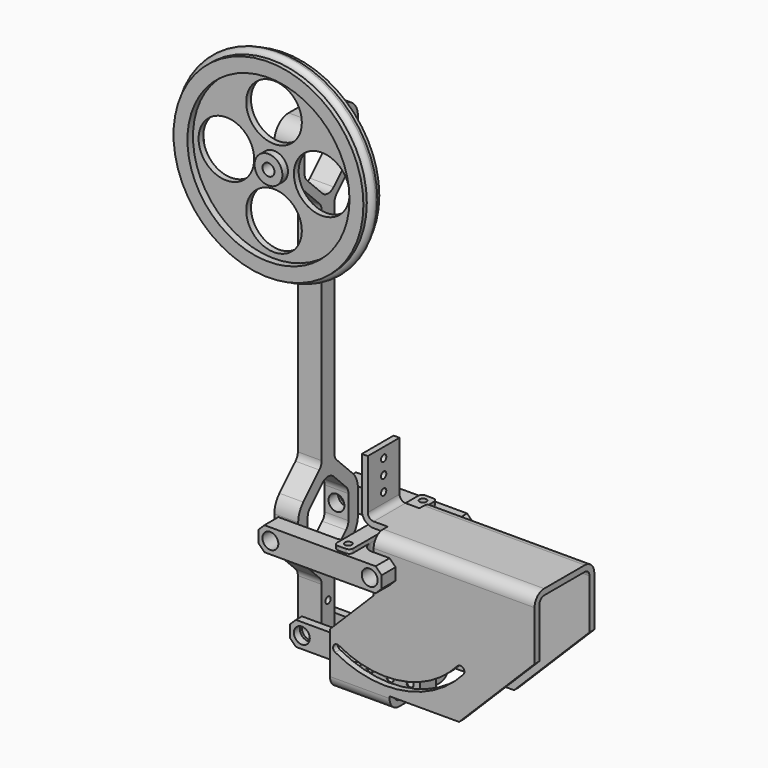
from build123d import *

# Parameters (mm, degrees)
F2_R           = 1.65
F3_DEPTH       = 6
F4_SIZE        = 3
F6_DEPTH       = 6
F7_SIZE        = 3
F10_DEPTH      = 6
F11_SIZE       = 3
F12_R          = 4
F13_DEPTH      = 28.801
F13_DEPTH_BACK = 28.801
F15_DEPTH      = 18.8
F16_T          = -3
F18_R          = 4
F19_DEPTH      = 47.601
F20_W          = 30
F20_H          = 15
F21_DEPTH      = 10
F22_R          = 3
F23_DEPTH      = 4.4
F24_R          = 1.65
F25_DEPTH      = 44.601
F26_R          = 2
F27_DEPTH      = 0.1
F28_R          = 2
F29_DEPTH      = 0.1
F30_R          = 2
F31_DEPTH      = 0.1
F32_R          = 6
F33_R          = 3
F36_R          = 14
F37_DEPTH      = 55.301
F38_R          = 1.25
F39_DEPTH      = 8
F38_R_2        = 1.5
F40_DEPTH      = 0.1
F41_R          = 1.5
F41_R_2        = 1.25
F42_DEPTH      = 0.1
F44_W          = 3
F44_H          = 28
F45_DEPTH      = 10
F46_R          = 1.75
F47_DEPTH      = 2
F48_R          = 6
F49_R          = 3
F50_R          = 1.65
F51_DEPTH      = 94.001
F53_DEPTH      = 30


# Not quite as in the source:
# - a feature names something its author has since deleted; it is built from what else it names


with BuildPart() as f3:
    # F2 (on Right) → F3 (new body, symmetric)
    with BuildSketch(Plane.YZ):
        with BuildLine():
            Line((5.4644660941, 141.9365440327), (16.1639610307, 152.6360389693))
            ThreePointArc((16.1639610307, 152.6360389693), (18.1149157926, 155.5558491087), (18.8, 159))
            Line((18.8, 159), (18.8, 171))
            ThreePointArc((18.8, 171), (16.1639610307, 177.3639610307), (9.8, 180))
            Line((9.8, 180), (0, 180))
            Line((0, 180), (-9.8, 180))
            ThreePointArc((-9.8, 180), (-16.1639610307, 177.3639610307), (-18.8, 171))
            Line((-18.8, 171), (-18.8, 159))
            ThreePointArc((-18.8, 159), (-18.1149157926, 155.5558491087), (-16.1639610307, 152.6360389693))
            Line((-16.1639610307, 152.6360389693), (-5.4644660941, 141.9365440327))
            ThreePointArc((-5.4644660941, 141.9365440327), (-4.3806023374, 140.3144272886), (-4, 138.4010101268))
            Line((-4, 138.4010101268), (-4, 27.427416998))
            ThreePointArc((-4, 27.427416998), (-4.3806023374, 25.5139998361), (-5.4644660941, 23.891883092))
            Line((-5.4644660941, 23.891883092), (-15.5781745931, 13.7781745931))
            ThreePointArc((-15.5781745931, 13.7781745931), (-17.9626748576, 10.209517756), (-18.8, 6))
            Line((-18.8, 6), (-18.8, -6))
            ThreePointArc((-18.8, -6), (-17.9626748576, -10.209517756), (-15.5781745931, -13.7781745931))
            Line((-15.5781745931, -13.7781745931), (-5.4644660941, -23.891883092))
            ThreePointArc((-5.4644660941, -23.891883092), (-4.3806023374, -25.5139998361), (-4, -27.427416998))
            Line((-4, -27.427416998), (-4, -50))
            Line((-4, -50), (-4, -56))
            Line((-4, -56), (0, -56))
            Line((0, -56), (4, -56))
            Line((4, -56), (4, -50))
            Line((4, -50), (4, -27.427416998))
            ThreePointArc((4, -27.427416998), (4.3806023374, -25.5139998361), (5.4644660941, -23.891883092))
            Line((5.4644660941, -23.891883092), (15.5781745931, -13.7781745931))
            ThreePointArc((15.5781745931, -13.7781745931), (17.9626748576, -10.209517756), (18.8, -6))
            Line((18.8, -6), (18.8, 6))
            ThreePointArc((18.8, 6), (17.9626748576, 10.209517756), (15.5781745931, 13.7781745931))
            Line((15.5781745931, 13.7781745931), (5.4644660941, 23.891883092))
            ThreePointArc((5.4644660941, 23.891883092), (4.3806023374, 25.5139998361), (4, 27.427416998))
            Line((4, 27.427416998), (4, 138.4010101268))
            ThreePointArc((4, 138.4010101268), (4.3806023374, 140.3144272886), (5.4644660941, 141.9365440327))
        make_face()
        with Locations((0, -36)):
            Circle(F2_R, mode=Mode.SUBTRACT)
        with BuildLine():
            ThreePointArc((-3.5355339059, 17.3355339059), (0, 18.8), (3.5355339059, 17.3355339059))
            Line((3.5355339059, 17.3355339059), (11.3355339059, 9.5355339059))
            ThreePointArc((11.3355339059, 9.5355339059), (12.4193976626, 7.9134171618), (12.8, 6))
            Line((12.8, 6), (12.8, -6))
            ThreePointArc((12.8, -6), (12.4193976626, -7.9134171618), (11.3355339059, -9.5355339059))
            Line((11.3355339059, -9.5355339059), (3.5355339059, -17.3355339059))
            ThreePointArc((3.5355339059, -17.3355339059), (0, -18.8), (-3.5355339059, -17.3355339059))
            Line((-3.5355339059, -17.3355339059), (-11.3355339059, -9.5355339059))
            ThreePointArc((-11.3355339059, -9.5355339059), (-12.4193976626, -7.9134171618), (-12.8, -6))
            Line((-12.8, -6), (-12.8, 6))
            ThreePointArc((-12.8, 6), (-12.4193976626, 7.9134171618), (-11.3355339059, 9.5355339059))
            Line((-11.3355339059, 9.5355339059), (-3.5355339059, 17.3355339059))
        make_face(mode=Mode.SUBTRACT)
        with BuildLine():
            ThreePointArc((14.8, 159), (14.4193976626, 157.0865828382), (13.3355339059, 155.4644660941))
            Line((13.3355339059, 155.4644660941), (3.5355339059, 145.6644660941))
            ThreePointArc((3.5355339059, 145.6644660941), (0, 144.2), (-3.5355339059, 145.6644660941))
            Line((-3.5355339059, 145.6644660941), (-13.3355339059, 155.4644660941))
            ThreePointArc((-13.3355339059, 155.4644660941), (-14.4193976626, 157.0865828382), (-14.8, 159))
            Line((-14.8, 159), (-14.8, 171))
            ThreePointArc((-14.8, 171), (-13.3355339059, 174.5355339059), (-9.8, 176))
            Line((-9.8, 176), (0, 176))
            Line((0, 176), (9.8, 176))
            ThreePointArc((9.8, 176), (13.3355339059, 174.5355339059), (14.8, 171))
            Line((14.8, 171), (14.8, 159))
        make_face(mode=Mode.SUBTRACT)
    extrude(amount=F3_DEPTH, both=True)

    # F4
    f4_edges = [f3.edges().sort_by_distance(p)[0] for p in [
        (6, 0, -56),
        (-6, 0, -56),
    ]]
    chamfer(f4_edges, length=F4_SIZE)


with BuildPart() as f6:
    # F5 (on Top) → F6 (new body, symmetric)
    with BuildSketch(Plane.XY):
        with BuildLine():
            Line((31, 28.8), (-6, 28.8))
            Line((-6, 28.8), (-6, 20))
            Line((-6, 20), (26, 20))
            ThreePointArc((26, 20), (29.5355339059, 18.5355339059), (31, 15))
            Line((31, 15), (31, 0))
            Line((31, 0), (31, -15))
            ThreePointArc((31, -15), (29.5355339059, -18.5355339059), (26, -20))
            Line((26, -20), (-6, -20))
            Line((-6, -20), (-6, -28.8))
            Line((-6, -28.8), (31, -28.8))
            Line((31, -28.8), (44, -28.8))
            Line((44, -28.8), (56, -28.8))
            Line((56, -28.8), (56, -20))
            Line((56, -20), (44, -20))
            ThreePointArc((44, -20), (40.4644660941, -18.5355339059), (39, -15))
            Line((39, -15), (39, 0))
            Line((39, 0), (39, 15))
            ThreePointArc((39, 15), (40.4644660941, 18.5355339059), (44, 20))
            Line((44, 20), (56, 20))
            Line((56, 20), (56, 28.8))
            Line((56, 28.8), (44, 28.8))
            Line((44, 28.8), (31, 28.8))
        make_face()
    extrude(amount=F6_DEPTH, both=True)

    # F7
    f7_edges = [f6.edges().sort_by_distance(p)[0] for p in [
        (56, -24.4, 6),
        (56, -24.4, -6),
        (56, 24.4, 6),
        (56, 24.4, -6),
        (-6, -24.4, 6),
        (-6, -24.4, -6),
        (-6, 24.4, 6),
        (-6, 24.4, -6),
    ]]
    chamfer(f7_edges, length=F7_SIZE)


with BuildPart() as f10:
    # F9 (on offset) → F10 (new body, symmetric)
    with BuildSketch(Plane.XY.offset(-50)):
        with BuildLine():
            Line((11, -5.2), (-6, -5.2))
            Line((-6, -5.2), (-6, -9))
            Line((-6, -9), (16, -9))
            ThreePointArc((16, -9), (17.9134171618, -8.6193976626), (19.5355339059, -7.5355339059))
            Line((19.5355339059, -7.5355339059), (21.6066017178, -5.4644660941))
            ThreePointArc((21.6066017178, -5.4644660941), (23.2287184619, -4.3806023374), (25.1421356237, -4))
            Line((25.1421356237, -4), (56, -4))
            Line((56, -4), (56, 0))
            Line((56, 0), (56, 4))
            Line((56, 4), (25.1421356237, 4))
            ThreePointArc((25.1421356237, 4), (23.2287184619, 4.3806023374), (21.6066017178, 5.4644660941))
            Line((21.6066017178, 5.4644660941), (19.5355339059, 7.5355339059))
            ThreePointArc((19.5355339059, 7.5355339059), (17.9134171618, 8.6193976626), (16, 9))
            Line((16, 9), (-6, 9))
            Line((-6, 9), (-6, 5.2))
            Line((-6, 5.2), (11, 5.2))
            ThreePointArc((11, 5.2), (14.5355339059, 3.7355339059), (16, 0.2))
            Line((16, 0.2), (16, 0))
            Line((16, 0), (16, -0.2))
            ThreePointArc((16, -0.2), (14.5355339059, -3.7355339059), (11, -5.2))
        make_face()
    extrude(amount=F10_DEPTH, both=True)

    # F11
    f11_edges = [f10.edges().sort_by_distance(p)[0] for p in [
        (-6, -7.1, -56),
        (-6, -7.1, -44),
        (-6, 7.1, -56),
        (-6, 7.1, -44),
        (56, 0, -56),
        (56, 0, -44),
    ]]
    chamfer(f11_edges, length=F11_SIZE)


with BuildPart() as f13_tool:
    # F12 (on Front) → F13 (new body, two sides)
    with BuildSketch(Plane.XZ) as f13_sk:
        Circle(F12_R)
        with Locations((0, -50)):
            Circle(F12_R)
        with Locations((0, 165)):
            Circle(F12_R)
        with Locations((50, 0)):
            Circle(F12_R)
        with Locations((50, -50)):
            Circle(F12_R)
    extrude(amount=-F13_DEPTH)
    extrude(f13_sk.sketch, amount=F13_DEPTH_BACK)


with BuildPart() as f3_1:
    add(f3.part)

    # F13: cut by f13_tool
    add(f13_tool.part, mode=Mode.SUBTRACT)


with BuildPart() as f6_1:
    add(f6.part)

    # F13: cut by f13_tool
    add(f13_tool.part, mode=Mode.SUBTRACT)

    # F38 (on face) → F39 (cut, through all)
    with BuildSketch(Plane(origin=(31, 0, 0), x_dir=(0, -1, 0), z_dir=(-1, 0, 0))):
        Circle(F38_R)
    extrude(amount=-F39_DEPTH, mode=Mode.SUBTRACT)

    # F38 (on face) → F40 (cut)
    with BuildSketch(Plane(origin=(31, 0, 0), x_dir=(0, -1, 0), z_dir=(-1, 0, 0))):
        Circle(F38_R_2)
        Circle(F38_R, mode=Mode.SUBTRACT)
    extrude(amount=-F40_DEPTH, mode=Mode.SUBTRACT)

    # F41 (on face) → F42 (cut)
    with BuildSketch(Plane.YZ.offset(39)):
        Circle(F41_R)
        Circle(F41_R_2, mode=Mode.SUBTRACT)
    extrude(amount=-F42_DEPTH, mode=Mode.SUBTRACT)


with BuildPart() as f10_1:
    add(f10.part)

    # F13: cut by f13_tool
    add(f13_tool.part, mode=Mode.SUBTRACT)


with BuildPart() as f15:
    # F14 (on Front) → F15 (new body, symmetric)
    with BuildSketch(Plane.XZ):
        Polygon((125, 13), (44, 13), (44, -14), (22, -36), (22, -56), (87, -56), (125, -18), align=None)
    extrude(amount=F15_DEPTH, both=True)

    # F16
    f16_openings = [f15.faces().sort_by_distance(p)[0] for p in [
        (54.5, 0, -56),
        (22, 0, -46),
        (33, 0, -25),
        (44, 0, -0.5),
        (125, 0, -2.5),
        (106, 0, -37),
    ]]
    offset(amount=F16_T, openings=f16_openings)

    # F18 (on face) → F19 (cut, through all)
    with BuildSketch(Plane.XZ.offset(18.8)):
        with BuildLine():
            ThreePointArc((26.6241816764, -41.8661392739), (23.8349009032, -42.6566535169), (24.6254151462, -45.4459342901))
            ThreePointArc((24.6254151462, -45.4459342901), (58.8887201904, -51.2854087765), (89.1884132047, -34.2559596347))
            ThreePointArc((89.1884132047, -34.2559596347), (88.9941475022, -31.3633378418), (86.1015257093, -31.5576035444))
            ThreePointArc((86.1015257093, -31.5576035444), (58.1885520294, -47.245635943), (26.6241816764, -41.8661392739))
        make_face()
        with Locations((50, 0)):
            Circle(F18_R)
    extrude(amount=-F19_DEPTH, mode=Mode.SUBTRACT)

    # F32
    f32_edges = [f15.edges().sort_by_distance(p)[0] for p in [
        (84.5, -18.8, 13),
        (84.5, 18.8, 13),
    ]]
    fillet(f32_edges, radius=F32_R)

    # F33
    f33_edges = [f15.edges().sort_by_distance(p)[0] for p in [
        (84.5, -15.8, 10),
        (84.5, 15.8, 10),
    ]]
    fillet(f33_edges, radius=F33_R)

    # F44 (on Front) → F45 (join, symmetric)
    with BuildSketch(Plane.XZ):
        Polygon((44, 10), (44, 13), (34, 13), (31, 13), (31, 10), align=None)
        with Locations((32.5, 27)):
            Rectangle(F44_W, F44_H)
    extrude(amount=F45_DEPTH, both=True)

    # F48
    f48_edges = [f15.edges().sort_by_distance(p)[0] for p in [
        (31, 0, 10),
    ]]
    fillet(f48_edges, radius=F48_R)

    # F49
    f49_edges = [f15.edges().sort_by_distance(p)[0] for p in [
        (34, 0, 13),
    ]]
    fillet(f49_edges, radius=F49_R)

    # F50 (on face) → F51 (cut, through all)
    with BuildSketch(Plane(origin=(31, 0, 0), x_dir=(0, -1, 0), z_dir=(-1, 0, 0))):
        with Locations((0, 21)):
            Circle(F50_R)
        with Locations((0, 28.5)):
            Circle(F50_R)
        with Locations((0, 36)):
            Circle(F50_R)
    extrude(amount=-F51_DEPTH, mode=Mode.SUBTRACT)

    # F52 (on face) → F53 (join)
    with BuildSketch(Plane(origin=(22, 0, 0), x_dir=(0, -1, 0), z_dir=(-1, 0, 0))):
        with BuildLine():
            Line((18.8, -57), (18.8, -56))
            Line((18.8, -56), (15.8, -56))
            Line((15.8, -56), (15.8, -57))
            ThreePointArc((15.8, -57), (14.9213203436, -59.1213203436), (12.8, -60))
            Line((12.8, -60), (1.8, -60))
            Line((1.8, -60), (1.8, -63))
            Line((1.8, -63), (12.8, -63))
            ThreePointArc((12.8, -63), (17.0426406871, -61.2426406871), (18.8, -57))
        make_face()
        with BuildLine():
            Line((-18.8, -56), (-18.8, -57))
            ThreePointArc((-18.8, -57), (-17.0426406871, -61.2426406871), (-12.8, -63))
            Line((-12.8, -63), (-1.8, -63))
            Line((-1.8, -63), (-1.8, -60))
            Line((-1.8, -60), (-12.8, -60))
            ThreePointArc((-12.8, -60), (-14.9213203436, -59.1213203436), (-15.8, -57))
            Line((-15.8, -57), (-15.8, -56))
            Line((-15.8, -56), (-18.8, -56))
        make_face()
    extrude(amount=-F53_DEPTH)


with BuildPart() as f21:
    # F20 (on face) → F21 (new body)
    with BuildSketch(Plane(origin=(0, -15.8, 0), x_dir=(-1, 0, 0), z_dir=(0, 1, 0))):
        with Locations((-50, -48.5)):
            Rectangle(F20_W, F20_H)
    extrude(amount=F21_DEPTH)

    # F22 (on face) → F23 (cut)
    with BuildSketch(Plane(origin=(0, -5.8, 0), x_dir=(-1, 0, 0), z_dir=(0, 1, 0))):
        with Locations((-50, -50)):
            Circle(F22_R)
    extrude(amount=-F23_DEPTH, mode=Mode.SUBTRACT)

    # F24 (on face) → F25 (cut, through all)
    with BuildSketch(Plane.XZ.offset(15.8)):
        with Locations((50, -50)):
            Circle(F24_R)
        with Locations((60, -49)):
            Circle(F24_R)
        with Locations((40, -49)):
            Circle(F24_R)
    extrude(amount=-F25_DEPTH, mode=Mode.SUBTRACT)

    # F26 (on face) → F27 (cut)
    with BuildSketch(Plane.XZ.offset(15.8)):
        with Locations((40, -49)):
            Circle(F26_R)
        with Locations((50, -50)):
            Circle(F26_R)
        with Locations((60, -49)):
            Circle(F26_R)
    extrude(amount=-F27_DEPTH, mode=Mode.SUBTRACT)

    # F28 (on face) → F29 (cut)
    with BuildSketch(Plane(origin=(0, -5.8, 0), x_dir=(-1, 0, 0), z_dir=(0, 1, 0))):
        with Locations((-60, -49)):
            Circle(F28_R)
        with Locations((-40, -49)):
            Circle(F28_R)
    extrude(amount=-F29_DEPTH, mode=Mode.SUBTRACT)

    # F30 (on face) → F31 (cut)
    with BuildSketch(Plane(origin=(0, -10.2, 0), x_dir=(-1, 0, 0), z_dir=(0, 1, 0))):
        with Locations((-50, -50)):
            Circle(F30_R)
    extrude(amount=-F31_DEPTH, mode=Mode.SUBTRACT)


with BuildPart() as f35:
    # F34 (on line) → F35 (revolve)
    with BuildSketch(Plane.XY.offset(165)):
        Polygon((7, -20), (3, -20), (3, -30), (7, -30), (7, -26.5), (40.8, -26.5), (40.8, -30), (47.8, -30), (47.8, -27.85), (47.15, -27.85), (44.3, -27.85), (44.3, -25), (44.3, -22.15), (47.15, -22.15), (47.8, -22.15), (47.8, -20), (40.8, -20), (40.8, -23.5), (7, -23.5), align=None)
        with BuildLine():
            ThreePointArc((50, -25), (49.1652543264, -22.9847456736), (47.15, -22.15))
            ThreePointArc((47.15, -22.15), (45.1347456736, -22.9847456736), (44.3, -25))
            ThreePointArc((44.3, -25), (45.1347456736, -27.0152543264), (47.15, -27.85))
            ThreePointArc((47.15, -27.85), (49.1652543264, -27.0152543264), (50, -25))
        make_face()
    revolve(axis=Axis((0, -25, 165), (0, -1, 0)))

    # F36 (on face) → F37 (cut, through all)
    with BuildSketch(Plane.XZ.offset(26.5)):
        with Locations((0, 189)):
            Circle(F36_R)
        with Locations((-24, 165)):
            Circle(F36_R)
        with Locations((0, 141)):
            Circle(F36_R)
        with Locations((24, 165)):
            Circle(F36_R)
    extrude(amount=-F37_DEPTH, mode=Mode.SUBTRACT)


with BuildPart() as f47:
    # F46 (on face) → F47 (new body)
    with BuildSketch(Plane.XY.offset(6)):
        with BuildLine():
            Line((37, 27.5), (33, 27.5))
            ThreePointArc((33, 27.5), (31.5857864376, 26.9142135624), (31, 25.5))
            Line((31, 25.5), (31, -25.5))
            ThreePointArc((31, -25.5), (31.5857864376, -26.9142135624), (33, -27.5))
            Line((33, -27.5), (37, -27.5))
            ThreePointArc((37, -27.5), (38.4142135624, -26.9142135624), (39, -25.5))
            Line((39, -25.5), (39, 25.5))
            ThreePointArc((39, 25.5), (38.4142135624, 26.9142135624), (37, 27.5))
        make_face()
        with Locations((35, -23.5)):
            Circle(F46_R, mode=Mode.SUBTRACT)
        with Locations((35, 23.5)):
            Circle(F46_R, mode=Mode.SUBTRACT)
    extrude(amount=F47_DEPTH)


solid = Compound([f3_1.part, f6_1.part, f10_1.part, f15.part, f21.part, f35.part, f47.part])
